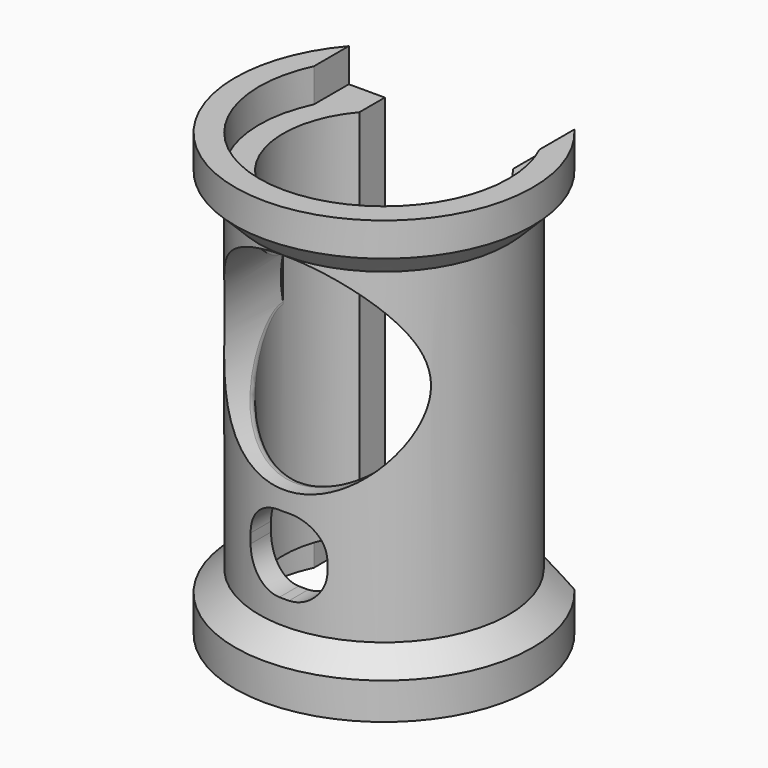
from build123d import *

# Parameters (mm, degrees)
F2_W      = 16
F2_H      = 12.7785220167
F3_DEPTH  = 46.001
F4_W      = 23.5
F4_H      = 13.4564294844
F5_DEPTH  = 3.5
F6_W      = 23.5
F6_H      = 13.0310004231
F7_DEPTH  = 3.8
F8_R      = 10.75
F9_DEPTH  = 25
F11_W     = 31.7701289256
F11_H     = 9.9966360929
F12_DEPTH = 46.001
F14_DEPTH = 25
F15_R     = 1


with BuildPart() as f1:
    # F0 (on Front) → F1 (revolve)
    with BuildSketch(Plane.XZ):
        Polygon((-15.5, 0), (-13, 0), (-13, 3.8), (-10.5, 3.8), (-10.5, 42.5), (-13, 42.5), (-13, 46), (-15.5, 46), (-15.5, 42.5), (-13, 40), (-13, 6), (-15.5, 3.8), align=None)
    revolve(axis=Axis((0, 0, 24.8965322971), (0, 0, 1)))

    # F2 (on face) → F3 (cut, through all)
    with BuildSketch(Plane.XY.offset(46)):
        with Locations((0, 11.7036290467)):
            Rectangle(F2_W, F2_H)
    extrude(amount=-F3_DEPTH, mode=Mode.SUBTRACT)

    # F4 (on face) → F5 (cut, through all)
    with BuildSketch(Plane.XY.offset(46)):
        with Locations((0, 10.8011863194)):
            Rectangle(F4_W, F4_H)
    extrude(amount=-F5_DEPTH, mode=Mode.SUBTRACT)

    # F6 (on face) → F7 (cut, through all)
    with BuildSketch(Plane(origin=(0, 0, 0), x_dir=(1, 0, 0), z_dir=(0, 0, -1))):
        with Locations((0, -9.3560743844)):
            Rectangle(F6_W, F6_H)
    extrude(amount=-F7_DEPTH, mode=Mode.SUBTRACT)

    # F8 (on Front) → F9 (cut)
    with BuildSketch(Plane.XZ):
        with Locations((0, 29.25)):
            Circle(F8_R)
    extrude(amount=F9_DEPTH, mode=Mode.SUBTRACT)

    # F11 (on Top) → F12 (cut, through all)
    with BuildSketch(Plane.XY):
        with Locations((0.0608135015, 15.107101356)):
            Rectangle(F11_W, F11_H)
    extrude(amount=F12_DEPTH, mode=Mode.SUBTRACT)

    # F13 (on Front) → F14 (cut)
    with BuildSketch(Plane.XZ):
        with BuildLine():
            Line((0.5, 16.5), (-0.5, 16.5))
            ThreePointArc((-0.5, 16.5), (-2.9748737342, 15.4748737342), (-4, 13))
            Line((-4, 13), (-4, 12))
            ThreePointArc((-4, 12), (-2.9748737342, 9.5251262658), (-0.5, 8.5))
            Line((-0.5, 8.5), (0.5, 8.5))
            ThreePointArc((0.5, 8.5), (2.9748737342, 9.5251262658), (4, 12))
            Line((4, 12), (4, 13))
            ThreePointArc((4, 13), (2.9748737342, 15.4748737342), (0.5, 16.5))
        make_face()
    extrude(amount=F14_DEPTH, mode=Mode.SUBTRACT)

    # F15
    f15_edges = [f1.edges().sort_by_distance(p)[0] for p in [
        (0.039521, -10.499926, 18.500073),
    ]]
    fillet(f15_edges, radius=F15_R)


solid = f1.part
